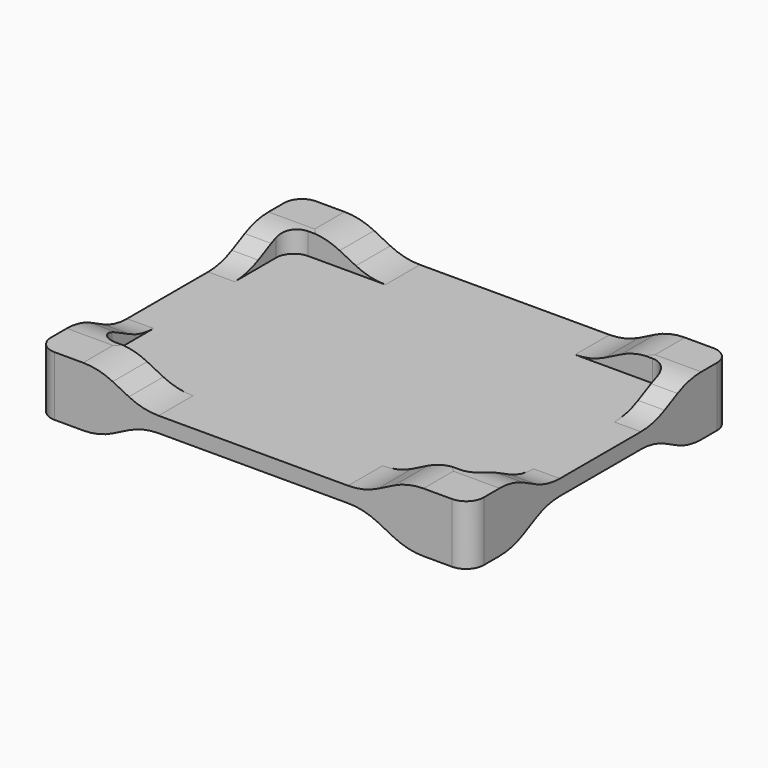
from build123d import *

# Parameters (mm, degrees)
F2_DEPTH      = 8.5
F2_DEPTH_BACK = 5
F3_DEPTH      = 5
F5_START      = -3.5
F5_DEPTH      = 5
F7_DEPTH      = 98.001
F9_DEPTH      = 74.001
F10_T1_DEPTH  = 6.0466451645
F10_T3_DEPTH  = 6
F10_T5_DEPTH  = 3.25
F10_T7_DEPTH  = 3.5113155246
F10_T9_DEPTH  = 6
F10_T11_DEPTH = 9.75
F10_T13_DEPTH = 9.75
F10_T15_DEPTH = 23.7050983125
F10_T17_DEPTH = 23.751743477
F10_T19_DEPTH = 21.2164138371
F10_T21_DEPTH = 20.9550983125
F10_T23_DEPTH = 24.10822467
F10_T25_DEPTH = 24.10822467
F10_T27_DEPTH = 27.4550983125
F10_T29_DEPTH = 27.4550983125


# Not quite as in the source:
# - a fillet or chamfer that OpenCascade refuses, or shapes differently, is made with other operations: its cross-section is extruded or revolved along the edge and cut away or added


with BuildPart() as f2:
    # F1 (on Top) → F2 (new body, two sides)
    with BuildSketch(Plane.XY) as f2_sk:
        with BuildLine():
            ThreePointArc((-6, -5.75), (-4.8284271247, -8.5784271247), (-2, -9.75))
            Line((-2, -9.75), (88, -9.75))
            ThreePointArc((88, -9.75), (90.8284271247, -8.5784271247), (92, -5.75))
            Line((92, -5.75), (92, 60.25))
            ThreePointArc((92, 60.25), (90.8284271247, 63.0784271247), (88, 64.25))
            Line((88, 64.25), (-2, 64.25))
            ThreePointArc((-2, 64.25), (-4.8284271247, 63.0784271247), (-6, 60.25))
            Line((-6, 60.25), (-6, -5.75))
        make_face()
    extrude(amount=-F2_DEPTH)
    extrude(f2_sk.sketch, amount=F2_DEPTH_BACK)

    # F0 (on Top) → F3 (cut)
    with BuildSketch(Plane.XY):
        with BuildLine():
            ThreePointArc((0, 4), (1.1715728753, 1.1715728753), (4, 0))
            Line((4, 0), (82, 0))
            ThreePointArc((82, 0), (84.8284271247, 1.1715728753), (86, 4))
            Line((86, 4), (86, 50.5))
            ThreePointArc((86, 50.5), (84.8284271247, 53.3284271247), (82, 54.5))
            Line((82, 54.5), (4, 54.5))
            ThreePointArc((4, 54.5), (1.1715728753, 53.3284271247), (0, 50.5))
            Line((0, 50.5), (0, 4))
        make_face()
    extrude(amount=F3_DEPTH, mode=Mode.SUBTRACT)

    # F4 (on Top) → F5 (cut)
    with BuildSketch(Plane.XY.offset(F5_START)):
        with BuildLine():
            ThreePointArc((0, -2.5), (1.1715728753, -5.3284271247), (4, -6.5))
            Line((4, -6.5), (81.9533548355, -6.5))
            ThreePointArc((81.9533548355, -6.5), (84.7817819603, -5.3284271247), (85.9533548355, -2.5))
            Line((85.9533548355, -2.5), (85.9533548355, 56.7386844754))
            ThreePointArc((85.9533548355, 56.7386844754), (84.7817819603, 59.5671116002), (81.9533548355, 60.7386844754))
            Line((81.9533548355, 60.7386844754), (4, 60.7386844754))
            ThreePointArc((4, 60.7386844754), (1.1715728753, 59.5671116002), (0, 56.7386844754))
            Line((0, 56.7386844754), (0, -2.5))
        make_face()
    extrude(amount=-F5_DEPTH, mode=Mode.SUBTRACT)

    # F6 (on face) → F7 (cut, through all)
    with BuildSketch(Plane(origin=(-6, 0, 0), x_dir=(0, -1, 0), z_dir=(-1, 0, 0))):
        Polygon((-27.25, -8.5), (-2.25, -8.5), (-12.25, -3.5), (-27.25, -3.5), (-42.25, -3.5), (-52.25, -8.5), align=None)
        Polygon((-12.25, 0), (-2.25, 5), (-27.25, 5), (-52.25, 5), (-42.25, 0), (-27.25, 0), align=None)
    extrude(amount=-F7_DEPTH, mode=Mode.SUBTRACT)

    # F8 (on face) → F9 (cut, through all)
    with BuildSketch(Plane.XZ.offset(9.75)):
        Polygon((18, -3.5), (8, -8.5), (78, -8.5), (68, -3.5), (43, -3.5), align=None)
        Polygon((78, 5), (8, 5), (18, 0), (43, 0), (68, 0), align=None)
    extrude(amount=-F9_DEPTH, mode=Mode.SUBTRACT)

    # F10: fillet of radius 15 on 32 edges, made by hand

    # F10_s2 → F10_t1 (join)
    with BuildSketch(Plane.YZ.offset(85.9533548355)):
        with BuildLine():
            ThreePointArc((38.7089803375, -3.5), (42.1552741457, -3.901265158), (45.41718427, -5.083592135))
            Line((45.41718427, -5.083592135), (42.25, -3.5))
            Line((42.25, -3.5), (38.7089803375, -3.5))
        make_face()
        with BuildLine():
            ThreePointArc((15.7910196625, -3.5), (12.3447258543, -3.901265158), (9.08281573, -5.083592135))
            Line((9.08281573, -5.083592135), (12.25, -3.5))
            Line((12.25, -3.5), (15.7910196625, -3.5))
        make_face()
    extrude(amount=F10_T1_DEPTH)

    # F10_s4 → F10_t3 (join)
    with BuildSketch(Plane.YZ.offset(-6)):
        with BuildLine():
            ThreePointArc((38.7089803375, -3.5), (42.1552741457, -3.901265158), (45.41718427, -5.083592135))
            Line((45.41718427, -5.083592135), (42.25, -3.5))
            Line((42.25, -3.5), (38.7089803375, -3.5))
        make_face()
        with BuildLine():
            ThreePointArc((9.08281573, -5.083592135), (12.3447258543, -3.901265158), (15.7910196625, -3.5))
            Line((15.7910196625, -3.5), (12.25, -3.5))
            Line((12.25, -3.5), (9.08281573, -5.083592135))
        make_face()
        with BuildLine():
            ThreePointArc((15.7910196625, 0), (12.3447258543, 0.401265158), (9.08281573, 1.583592135))
            Line((9.08281573, 1.583592135), (12.25, 0))
            Line((12.25, 0), (15.7910196625, 0))
        make_face()
        with BuildLine():
            ThreePointArc((45.41718427, 1.583592135), (42.1552741457, 0.401265158), (38.7089803375, 0))
            Line((38.7089803375, 0), (42.25, 0))
            Line((42.25, 0), (45.41718427, 1.583592135))
        make_face()
    extrude(amount=F10_T3_DEPTH)

    # F10_s6 → F10_t5 (join)
    with BuildSketch(Plane.XZ.offset(6.5)):
        with BuildLine():
            ThreePointArc((64.4589803375, -3.5), (67.9052741457, -3.901265158), (71.16718427, -5.083592135))
            Line((71.16718427, -5.083592135), (68, -3.5))
            Line((68, -3.5), (64.4589803375, -3.5))
        make_face()
        with BuildLine():
            ThreePointArc((21.5410196625, -3.5), (18.0947258543, -3.901265158), (14.83281573, -5.083592135))
            Line((14.83281573, -5.083592135), (18, -3.5))
            Line((18, -3.5), (21.5410196625, -3.5))
        make_face()
    extrude(amount=F10_T5_DEPTH)

    # F10_s8 → F10_t7 (join)
    with BuildSketch(Plane.XZ.offset(-64.25)):
        with BuildLine():
            ThreePointArc((64.4589803375, -3.5), (67.9052741457, -3.901265158), (71.16718427, -5.083592135))
            Line((71.16718427, -5.083592135), (68, -3.5))
            Line((68, -3.5), (64.4589803375, -3.5))
        make_face()
        with BuildLine():
            ThreePointArc((21.5410196625, -3.5), (18.0947258543, -3.901265158), (14.83281573, -5.083592135))
            Line((14.83281573, -5.083592135), (18, -3.5))
            Line((18, -3.5), (21.5410196625, -3.5))
        make_face()
    extrude(amount=F10_T7_DEPTH)

    # F10_s10 → F10_t9 (join)
    with BuildSketch(Plane.YZ.offset(86)):
        with BuildLine():
            ThreePointArc((15.7910196625, 0), (12.3447258543, 0.401265158), (9.08281573, 1.583592135))
            Line((9.08281573, 1.583592135), (12.25, 0))
            Line((12.25, 0), (15.7910196625, 0))
        make_face()
        with BuildLine():
            ThreePointArc((38.7089803375, 0), (42.1552741457, 0.401265158), (45.41718427, 1.583592135))
            Line((45.41718427, 1.583592135), (42.25, 0))
            Line((42.25, 0), (38.7089803375, 0))
        make_face()
    extrude(amount=F10_T9_DEPTH)

    # F10_s12 → F10_t11 (join)
    with BuildSketch(Plane.XZ.offset(-64.25)):
        with BuildLine():
            ThreePointArc((64.4589803375, 0), (67.9052741457, 0.401265158), (71.16718427, 1.583592135))
            Line((71.16718427, 1.583592135), (68, 0))
            Line((68, 0), (64.4589803375, 0))
        make_face()
        with BuildLine():
            ThreePointArc((21.5410196625, 0), (18.0947258543, 0.401265158), (14.83281573, 1.583592135))
            Line((14.83281573, 1.583592135), (18, 0))
            Line((18, 0), (21.5410196625, 0))
        make_face()
    extrude(amount=F10_T11_DEPTH)

    # F10_s14 → F10_t13 (join)
    with BuildSketch(Plane.XZ):
        with BuildLine():
            ThreePointArc((64.4589803375, 0), (67.9052741457, 0.401265158), (71.16718427, 1.583592135))
            Line((71.16718427, 1.583592135), (68, 0))
            Line((68, 0), (64.4589803375, 0))
        make_face()
        with BuildLine():
            ThreePointArc((21.5410196625, 0), (18.0947258543, 0.401265158), (14.83281573, 1.583592135))
            Line((14.83281573, 1.583592135), (18, 0))
            Line((18, 0), (21.5410196625, 0))
        make_face()
    extrude(amount=F10_T13_DEPTH)

    # F10_s16 → F10_t15 (cut)
    with BuildSketch(Plane.YZ.offset(-14.8525491562)):
        with BuildLine():
            ThreePointArc((-1.2910196625, -8.5), (2.1552741457, -8.098734842), (5.41718427, -6.916407865))
            Line((5.41718427, -6.916407865), (2.25, -8.5))
            Line((2.25, -8.5), (-1.2910196625, -8.5))
        make_face()
        with BuildLine():
            ThreePointArc((49.08281573, -6.916407865), (52.3447258543, -8.098734842), (55.7910196625, -8.5))
            Line((55.7910196625, -8.5), (52.25, -8.5))
            Line((52.25, -8.5), (49.08281573, -6.916407865))
        make_face()
    extrude(amount=F10_T15_DEPTH, mode=Mode.SUBTRACT)

    # F10_s18 → F10_t17 (cut)
    with BuildSketch(Plane.YZ.offset(77.1008056793)):
        with BuildLine():
            ThreePointArc((5.41718427, -6.916407865), (2.1552741457, -8.098734842), (-1.2910196625, -8.5))
            Line((-1.2910196625, -8.5), (2.25, -8.5))
            Line((2.25, -8.5), (5.41718427, -6.916407865))
        make_face()
        with BuildLine():
            ThreePointArc((49.08281573, -6.916407865), (52.3447258543, -8.098734842), (55.7910196625, -8.5))
            Line((55.7910196625, -8.5), (52.25, -8.5))
            Line((52.25, -8.5), (49.08281573, -6.916407865))
        make_face()
    extrude(amount=F10_T17_DEPTH, mode=Mode.SUBTRACT)

    # F10_s20 → F10_t19 (cut)
    with BuildSketch(Plane.XZ.offset(-73.1025491562)):
        with BuildLine():
            ThreePointArc((74.83281573, -6.916407865), (78.0947258543, -8.098734842), (81.5410196625, -8.5))
            Line((81.5410196625, -8.5), (78, -8.5))
            Line((78, -8.5), (74.83281573, -6.916407865))
        make_face()
        with BuildLine():
            ThreePointArc((11.16718427, -6.916407865), (7.9052741457, -8.098734842), (4.4589803375, -8.5))
            Line((4.4589803375, -8.5), (8, -8.5))
            Line((8, -8.5), (11.16718427, -6.916407865))
        make_face()
    extrude(amount=F10_T19_DEPTH, mode=Mode.SUBTRACT)

    # F10_s22 → F10_t21 (cut)
    with BuildSketch(Plane.XZ.offset(-2.3525491562)):
        with BuildLine():
            ThreePointArc((74.83281573, -6.916407865), (78.0947258543, -8.098734842), (81.5410196625, -8.5))
            Line((81.5410196625, -8.5), (78, -8.5))
            Line((78, -8.5), (74.83281573, -6.916407865))
        make_face()
        with BuildLine():
            ThreePointArc((11.16718427, -6.916407865), (7.9052741457, -8.098734842), (4.4589803375, -8.5))
            Line((4.4589803375, -8.5), (8, -8.5))
            Line((8, -8.5), (11.16718427, -6.916407865))
        make_face()
    extrude(amount=F10_T21_DEPTH, mode=Mode.SUBTRACT)

    # F10_s24 → F10_t23 (cut)
    with BuildSketch(Plane.YZ.offset(-14.8525491562)):
        with BuildLine():
            ThreePointArc((5.41718427, 3.416407865), (2.1552741457, 4.598734842), (-1.2910196625, 5))
            Line((-1.2910196625, 5), (2.25, 5))
            Line((2.25, 5), (5.41718427, 3.416407865))
        make_face()
        with BuildLine():
            ThreePointArc((55.7910196625, 5), (52.3447258543, 4.598734842), (49.08281573, 3.416407865))
            Line((49.08281573, 3.416407865), (52.25, 5))
            Line((52.25, 5), (55.7910196625, 5))
        make_face()
    extrude(amount=F10_T23_DEPTH, mode=Mode.SUBTRACT)

    # F10_s26 → F10_t25 (cut)
    with BuildSketch(Plane.YZ.offset(76.7443244862)):
        with BuildLine():
            ThreePointArc((-1.2910196625, 5), (2.1552741457, 4.598734842), (5.41718427, 3.416407865))
            Line((5.41718427, 3.416407865), (2.25, 5))
            Line((2.25, 5), (-1.2910196625, 5))
        make_face()
        with BuildLine():
            ThreePointArc((55.7910196625, 5), (52.3447258543, 4.598734842), (49.08281573, 3.416407865))
            Line((49.08281573, 3.416407865), (52.25, 5))
            Line((52.25, 5), (55.7910196625, 5))
        make_face()
    extrude(amount=F10_T25_DEPTH, mode=Mode.SUBTRACT)

    # F10_s28 → F10_t27 (cut)
    with BuildSketch(Plane.XZ.offset(-73.1025491562)):
        with BuildLine():
            ThreePointArc((81.5410196625, 5), (78.0947258543, 4.598734842), (74.83281573, 3.416407865))
            Line((74.83281573, 3.416407865), (78, 5))
            Line((78, 5), (81.5410196625, 5))
        make_face()
        with BuildLine():
            ThreePointArc((4.4589803375, 5), (7.9052741457, 4.598734842), (11.16718427, 3.416407865))
            Line((11.16718427, 3.416407865), (8, 5))
            Line((8, 5), (4.4589803375, 5))
        make_face()
    extrude(amount=F10_T27_DEPTH, mode=Mode.SUBTRACT)

    # F10_s30 → F10_t29 (cut)
    with BuildSketch(Plane.XZ.offset(-8.8525491562)):
        with BuildLine():
            ThreePointArc((81.5410196625, 5), (78.0947258543, 4.598734842), (74.83281573, 3.416407865))
            Line((74.83281573, 3.416407865), (78, 5))
            Line((78, 5), (81.5410196625, 5))
        make_face()
        with BuildLine():
            ThreePointArc((11.16718427, 3.416407865), (7.9052741457, 4.598734842), (4.4589803375, 5))
            Line((4.4589803375, 5), (8, 5))
            Line((8, 5), (11.16718427, 3.416407865))
        make_face()
    extrude(amount=F10_T29_DEPTH, mode=Mode.SUBTRACT)


solid = f2.part
